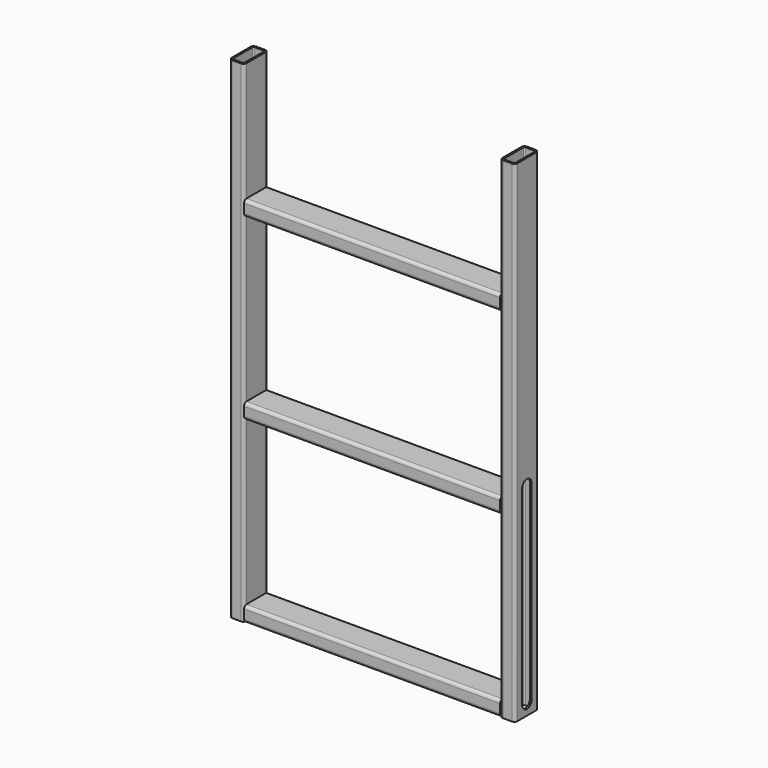
from build123d import *

# Parameters (mm, degrees)
F1_DEPTH = 825
F3_DEPTH = 3
F5_DEPTH = 430
F6_DEPTH = 430
F7_DEPTH = 430


# Not quite as in the source:
# - ends of sketch curves that miss each other by under 0.0002 mm in the source are joined


with BuildPart() as f1:
    # F0 (on Top) → F1 (new body)
    with BuildSketch(Plane.XY):
        with BuildLine():
            ThreePointArc((7.4849684764, -25.0075174148), (11.0205023823, -23.5430513207), (12.4849684764, -20.0075174148))
            Line((12.4849684764, -20.0075174148), (12.4849684764, 19.9924825852))
            ThreePointArc((12.4849684764, 19.9924825852), (11.0205023823, 23.5280164911), (7.4849684764, 24.9924825852))
            Line((7.4849684764, 24.9924825852), (-7.5150315236, 24.9924825852))
            ThreePointArc((-7.5150315236, 24.9924825852), (-11.0505654295, 23.5280164911), (-12.5150315236, 19.9924825852))
            Line((-12.5150315236, 19.9924825852), (-12.5150315236, -20.0075174148))
            ThreePointArc((-12.5150315236, -20.0075174148), (-11.0505654295, -23.5430513207), (-7.5150315236, -25.0075174148))
            Line((-7.5150315236, -25.0075174148), (7.4849684764, -25.0075174148))
        make_face()
        with BuildLine():
            Line((-7.5150315236, 21.9924825852), (7.4849684764, 21.9924825852))
            ThreePointArc((7.4849684764, 21.9924825852), (8.8991820388, 21.4066961476), (9.4849684764, 19.9924825852))
            Line((9.4849684764, 19.9924825852), (9.4849684764, -20.0075174148))
            ThreePointArc((9.4849684764, -20.0075174148), (8.8991820388, -21.4217309772), (7.4849684764, -22.0075174148))
            Line((7.4849684764, -22.0075174148), (-7.5150315236, -22.0075174148))
            ThreePointArc((-7.5150315236, -22.0075174148), (-8.929245086, -21.4217309772), (-9.5150315236, -20.0075174148))
            Line((-9.5150315236, -20.0075174148), (-9.5150315236, 19.9924825852))
            ThreePointArc((-9.5150315236, 19.9924825852), (-8.929245086, 21.4066961476), (-7.5150315236, 21.9924825852))
        make_face(mode=Mode.SUBTRACT)
    extrude(amount=F1_DEPTH)

    # F2 (on face) → F3 (cut)
    with BuildSketch(Plane(origin=(-12.5150315236, 0, 0), x_dir=(0, -1, 0), z_dir=(-1, 0, 0))):
        with BuildLine():
            Line((10, 20), (10, 340))
            ThreePointArc((10, 340), (0, 350), (-10, 340))
            Line((-10, 340), (-10, 20))
            ThreePointArc((-10, 20), (0, 10), (10, 20))
        make_face()
    extrude(amount=-F3_DEPTH, mode=Mode.SUBTRACT)


with BuildPart() as f5:
    # F4 (on face) → F5 (new body)
    with BuildSketch(Plane.YZ.offset(12.4849684764)):
        with BuildLine():
            Line((19.9924825852, 22), (19.9924825852, 25))
            Line((19.9924825852, 25), (-20, 25))
            ThreePointArc((-20, 25), (-20.0037587085, 24.9999985872), (-20.0075174148, 24.9999943488))
            Line((-20.0075174148, 24.9999943488), (-20.0075174148, 21.9999858721))
            ThreePointArc((-20.0075174148, 21.9999858721), (-20.003758714, 21.999996468), (-20, 22))
            Line((-20, 22), (19.9924825852, 22))
        make_face()
        with BuildLine():
            Line((19.9924825852, 0), (19.9924825852, 3))
            Line((19.9924825852, 3), (-20, 3))
            ThreePointArc((-20, 3), (-20.003758714, 3.000003532), (-20.0075174148, 3.0000141279))
            Line((-20.0075174148, 3.0000141279), (-20.0075174148, 0))
            ThreePointArc((-20.0075174148, 0), (-20.0037587042, 1.4128e-06), (-20, 0))
            Line((-20, 0), (19.9924825852, 0))
        make_face()
        with BuildLine():
            Line((-20.0075174148, 21.9999858721), (-20.0075174148, 24.9999943488))
            ThreePointArc((-20.0075174148, 24.9999943488), (-23.5381907152, 23.5328750987), (-25, 20))
            Line((-25, 20), (-25, 5))
            ThreePointArc((-25, 5), (-23.5381907122, 1.4671248983), (-20.0075174063, 5.6511e-06))
            Line((-20.0075174063, 5.6511e-06), (-20.0075174148, 3.0000141279))
            ThreePointArc((-20.0075174148, 3.0000141279), (-21.4168688771, 3.5884467473), (-22, 5))
            Line((-22, 5), (-22, 20))
            ThreePointArc((-22, 20), (-21.4168688771, 21.4115532527), (-20.0075174148, 21.9999858721))
        make_face()
        with BuildLine():
            Line((20, 25), (19.9924825852, 25))
            Line((19.9924825852, 25), (19.9924825852, 22))
            Line((19.9924825852, 22), (20, 22))
            ThreePointArc((20, 22), (21.4142135624, 21.4142135624), (22, 20))
            Line((22, 20), (22, 5))
            ThreePointArc((22, 5), (21.4142135624, 3.5857864376), (20, 3))
            Line((20, 3), (19.9924825852, 3))
            Line((19.9924825852, 3), (19.9924825852, 0))
            Line((19.9924825852, 0), (20, 0))
            ThreePointArc((20, 0), (23.5355339059, 1.4644660941), (25, 5))
            Line((25, 5), (25, 20))
            ThreePointArc((25, 20), (23.5355339059, 23.5355339059), (20, 25))
        make_face()
    extrude(amount=F5_DEPTH)


with BuildPart() as f6:
    # F4 (on face) → F6 (new body)
    with BuildSketch(Plane.YZ.offset(12.4849684764)):
        with BuildLine():
            Line((19.9924825852, 322), (19.9924825852, 325))
            Line((19.9924825852, 325), (-20, 325))
            ThreePointArc((-20, 325), (-20.0037587085, 324.9999985872), (-20.0075174148, 324.9999943488))
            Line((-20.0075174148, 324.9999943488), (-20.0075174148, 321.9999858721))
            ThreePointArc((-20.0075174148, 321.9999858721), (-20.003758714, 321.999996468), (-20, 322))
            Line((-20, 322), (19.9924825852, 322))
        make_face()
        with BuildLine():
            Line((20, 325), (19.9924825852, 325))
            Line((19.9924825852, 325), (19.9924825852, 322))
            Line((19.9924825852, 322), (20, 322))
            ThreePointArc((20, 322), (21.4142135624, 321.4142135624), (22, 320))
            Line((22, 320), (22, 305))
            ThreePointArc((22, 305), (21.4142135624, 303.5857864376), (20, 303))
            Line((20, 303), (19.9924825852, 303))
            Line((19.9924825852, 303), (19.9924825852, 300))
            Line((19.9924825852, 300), (20, 300))
            ThreePointArc((20, 300), (23.5355339059, 301.4644660941), (25, 305))
            Line((25, 305), (25, 320))
            ThreePointArc((25, 320), (23.5355339059, 323.5355339059), (20, 325))
        make_face()
        with BuildLine():
            Line((19.9924825852, 300), (19.9924825852, 303))
            Line((19.9924825852, 303), (-20, 303))
            ThreePointArc((-20, 303), (-20.003758714, 303.000003532), (-20.0075174148, 303.0000141279))
            Line((-20.0075174148, 303.0000141279), (-20.0075174148, 300.0000056512))
            ThreePointArc((-20.0075174148, 300.0000056512), (-20.0037587085, 300.0000014128), (-20, 300))
            Line((-20, 300), (19.9924825852, 300))
        make_face()
        with BuildLine():
            Line((-20.0075174148, 321.9999858721), (-20.0075174148, 324.9999943488))
            ThreePointArc((-20.0075174148, 324.9999943488), (-23.5381907152, 323.5328750987), (-25, 320))
            Line((-25, 320), (-25, 305))
            ThreePointArc((-25, 305), (-23.5381907152, 301.4671249013), (-20.0075174148, 300.0000056512))
            Line((-20.0075174148, 300.0000056512), (-20.0075174148, 303.0000141279))
            ThreePointArc((-20.0075174148, 303.0000141279), (-21.4168688771, 303.5884467473), (-22, 305))
            Line((-22, 305), (-22, 320))
            ThreePointArc((-22, 320), (-21.4168688771, 321.4115532527), (-20.0075174148, 321.9999858721))
        make_face()
    extrude(amount=F6_DEPTH)


with BuildPart() as f7:
    # F4 (on face) → F7 (new body)
    with BuildSketch(Plane.YZ.offset(12.4849684764)):
        with BuildLine():
            Line((-20.0075174148, 621.9999858721), (-20.0075174148, 624.9999943488))
            ThreePointArc((-20.0075174148, 624.9999943488), (-23.5381907152, 623.5328750987), (-25, 620))
            Line((-25, 620), (-25, 605))
            ThreePointArc((-25, 605), (-23.5381907152, 601.4671249013), (-20.0075174148, 600.0000056512))
            Line((-20.0075174148, 600.0000056512), (-20.0075174148, 603.0000141279))
            ThreePointArc((-20.0075174148, 603.0000141279), (-21.4168688771, 603.5884467473), (-22, 605))
            Line((-22, 605), (-22, 620))
            ThreePointArc((-22, 620), (-21.4168688771, 621.4115532527), (-20.0075174148, 621.9999858721))
        make_face()
        with BuildLine():
            Line((19.9924825852, 600), (19.9924825852, 603))
            Line((19.9924825852, 603), (-20, 603))
            ThreePointArc((-20, 603), (-20.003758714, 603.000003532), (-20.0075174148, 603.0000141279))
            Line((-20.0075174148, 603.0000141279), (-20.0075174148, 600.0000056512))
            ThreePointArc((-20.0075174148, 600.0000056512), (-20.0037587085, 600.0000014128), (-20, 600))
            Line((-20, 600), (19.9924825852, 600))
        make_face()
        with BuildLine():
            ThreePointArc((25, 620), (23.5355339059, 623.5355339059), (20, 625))
            Line((20, 625), (19.9924825852, 625))
            Line((19.9924825852, 625), (19.9924825852, 622))
            Line((19.9924825852, 622), (20, 622))
            ThreePointArc((20, 622), (21.4142135624, 621.4142135624), (22, 620))
            Line((22, 620), (22, 605))
            ThreePointArc((22, 605), (21.4142135624, 603.5857864376), (20, 603))
            Line((20, 603), (19.9924825852, 603))
            Line((19.9924825852, 603), (19.9924825852, 600))
            Line((19.9924825852, 600), (20, 600))
            ThreePointArc((20, 600), (23.5355339059, 601.4644660941), (25, 605))
            Line((25, 605), (25, 620))
        make_face()
        with BuildLine():
            Line((19.9924825852, 622), (19.9924825852, 625))
            Line((19.9924825852, 625), (-20, 625))
            ThreePointArc((-20, 625), (-20.0037587085, 624.9999985872), (-20.0075174148, 624.9999943488))
            Line((-20.0075174148, 624.9999943488), (-20.0075174148, 621.9999858721))
            ThreePointArc((-20.0075174148, 621.9999858721), (-20.003758714, 621.999996468), (-20, 622))
            Line((-20, 622), (19.9924825852, 622))
        make_face()
    extrude(amount=F7_DEPTH)


with BuildPart() as f8_1:
    # F8: instance of F1
    add(f1.part.mirror(Plane(origin=(12.4849684764, -0.0075174148, 412.5), x_dir=(0, 1, 0), z_dir=(1, 0, 0))))


with BuildPart() as f8_1_1:
    # F9: moved
    add(f8_1.part.moved(Location((430, 0, 0))))


solid = Compound([f1.part, f5.part, f6.part, f7.part, f8_1_1.part])
